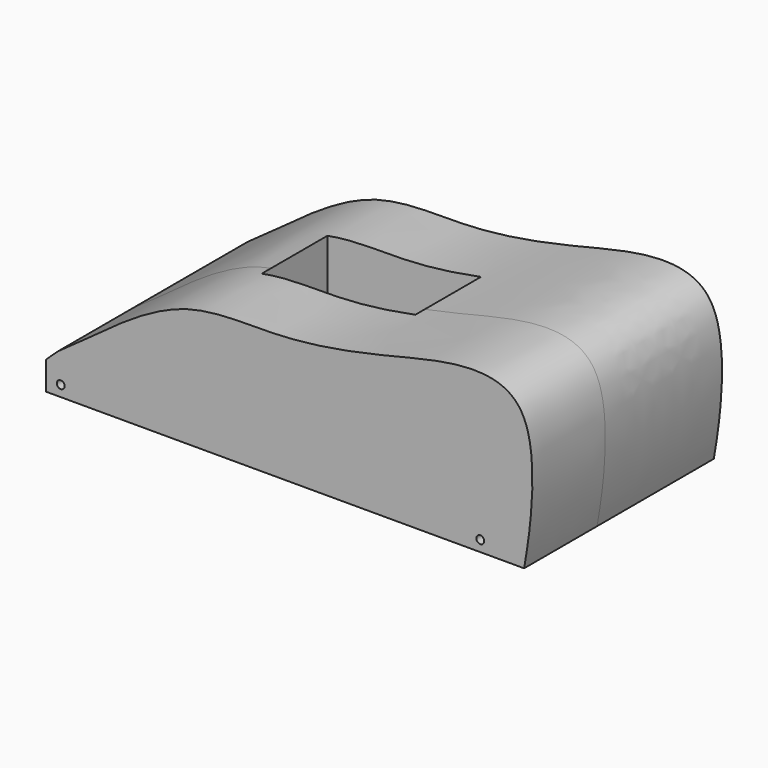
from build123d import *

# Parameters (mm, degrees)
F0_R     = 1.075
F1_DEPTH = 40
F2_DEPTH = 25
F3_DEPTH = 65.0010001
F5_W     = 42.0936179509
F5_H     = 22.4716748974
F6_DEPTH = 40.4


# Not quite as in the source:
# - a feature names something its author has since deleted; it is built from what else it names


with BuildPart() as f1:
    # F0 (on Front) → F1 (new body)
    with BuildSketch(Plane.XZ):
        with BuildLine():
            add(Edge.make_bspline(
                [(-59.500822073, 14.2913783373), (-56.6408981002, 16.2758116459), (-50.3327268236, 20.6972197265), (-26.2112339189, 39.1341727928), (0.9123679388, 36.7351149169), (29.2581893858, 41.4607157621), (78.5918665024, 55.8092687145), (68.6338635649, 5.7447523544), (68.2987782308, 3.4644304492)],
                knots=[0, 0, 0, 0, 0.1037500168, 0.2704106474, 0.4297306838, 0.6063016403, 0.793211467, 0.984487029, 0.984487029, 0.984487029, 0.984487029], degree=3))
            add(Edge.make_bspline(
                [(-59.500822073, 14.2913783373), (-60.6397116048, 13.241840497), (-61.7786011366, 12.1923026567), (-62.7701834043, 11.2554590394)],
                knots=[0, 0, 0, 0, 0.2457457998, 0.2457457998, 0.2457457998, 0.2457457998], degree=3))
            Line((-62.7701834043, 11.2554590394), (-62.7701834043, 3.4644304492))
            Line((-62.7701834043, 3.4644304492), (56.2773359432, 3.4644304492))
            Line((56.2773359432, 3.4644304492), (68.2987782308, 3.4644304492))
        make_face()
        with Locations((-58.7591566145, 6.4644304492)):
            Circle(F0_R, mode=Mode.SUBTRACT)
        with BuildLine():
            ThreePointArc((57.3523359432, 6.4644304492), (57.0374757329, 5.7042906594), (56.2773359432, 5.3894304492))
            ThreePointArc((56.2773359432, 5.3894304492), (55.5171961534, 7.2245702389), (57.3523359432, 6.4644304492))
        make_face(mode=Mode.SUBTRACT)
    extrude(amount=F1_DEPTH)

    # F2 (add): a face of the model
    f2_faces = [f1.faces().sort_by_distance(p)[0] for p in [
        (12.7289792957, -40, 21.2534595653),
    ]]
    extrude(f2_faces, amount=F2_DEPTH)

    # F0 (on Front) → F3 (cut, through all)
    with BuildSketch(Plane.XZ):
        with Locations((-58.7591566145, 6.4644304492)):
            Circle(F0_R)
    extrude(amount=F3_DEPTH, mode=Mode.SUBTRACT)

    # F5 (on offset) → F6 (cut)
    with BuildSketch(Plane.XY.offset(50.9)):
        with Locations((0, -32)):
            Rectangle(F5_W, F5_H)
    extrude(amount=-F6_DEPTH, mode=Mode.SUBTRACT)


solid = f1.part
